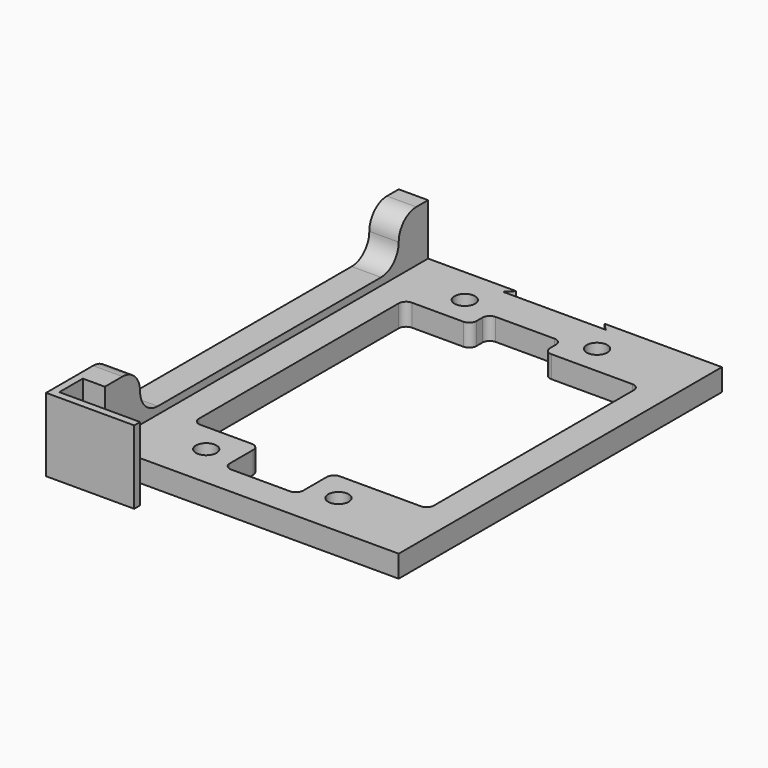
from build123d import *

# Parameters (mm, degrees)
F0_R     = 7
F1_DEPTH = 15
F2_DEPTH = 50
F3_W     = 220
F3_H     = 30
F4_DEPTH = 25
F5_R     = 14.99999
F6_R     = 5


# Not quite as in the source:
# - a fillet or chamfer is up to 0.001 mm smaller than in the source, because OpenCascade refuses the exact size


with BuildPart() as f1:
    # F0 (on Top) → F1 (new body)
    with BuildSketch(Plane.XY):
        Polygon((0, 300), (0, 0), (60, 0), (60, 5), (5, 5), (5, 25), (20, 25), (20, 300), align=None)
        Polygon((80, 300), (20, 300), (20, 25), (220, 25), (220, 300), (140, 300), (145, 295), (75, 295), align=None)
        with Locations((65, 55)):
            Circle(F0_R, mode=Mode.SUBTRACT)
        with Locations((155, 55)):
            Circle(F0_R, mode=Mode.SUBTRACT)
        Polygon((40, 75), (40, 255), (85, 255), (85, 270), (135, 270), (135, 255), (200, 255), (200, 75), (135, 75), (135, 45), (85, 45), (85, 75), align=None, mode=Mode.SUBTRACT)
        with Locations((65, 275)):
            Circle(F0_R, mode=Mode.SUBTRACT)
        with Locations((155, 275)):
            Circle(F0_R, mode=Mode.SUBTRACT)
    extrude(amount=F1_DEPTH)

    # F0 (on Top) → F2 (join)
    with BuildSketch(Plane.XY):
        Polygon((0, 300), (0, 0), (60, 0), (60, 5), (5, 5), (5, 25), (20, 25), (20, 300), align=None)
    extrude(amount=F2_DEPTH)

    # F3 (on face) → F4 (cut)
    with BuildSketch(Plane.YZ.offset(20)):
        with Locations((165, 35)):
            Rectangle(F3_W, F3_H)
    extrude(amount=-F4_DEPTH, mode=Mode.SUBTRACT)

    # F5 (radius 15 in the source; OpenCascade refuses exactly that, so slightly less here)
    f5_edges = [f1.edges().sort_by_distance(p)[0] for p in [
        (10, 275, 20),
        (10, 55, 20),
        (10, 275, 50),
        (10, 55, 50),
    ]]
    fillet(f5_edges, radius=F5_R)

    # F6
    f6_edges = [f1.edges().sort_by_distance(p)[0] for p in [
        (85, 75, 7.5),
        (135, 75, 7.5),
        (85, 45, 7.5),
        (135, 45, 7.5),
        (85, 255, 7.5),
        (85, 270, 7.5),
        (135, 255, 7.5),
        (135, 270, 7.5),
        (40, 75, 7.5),
        (40, 255, 7.5),
        (200, 255, 7.5),
        (200, 75, 7.5),
    ]]
    fillet(f6_edges, radius=F6_R)


solid = f1.part
